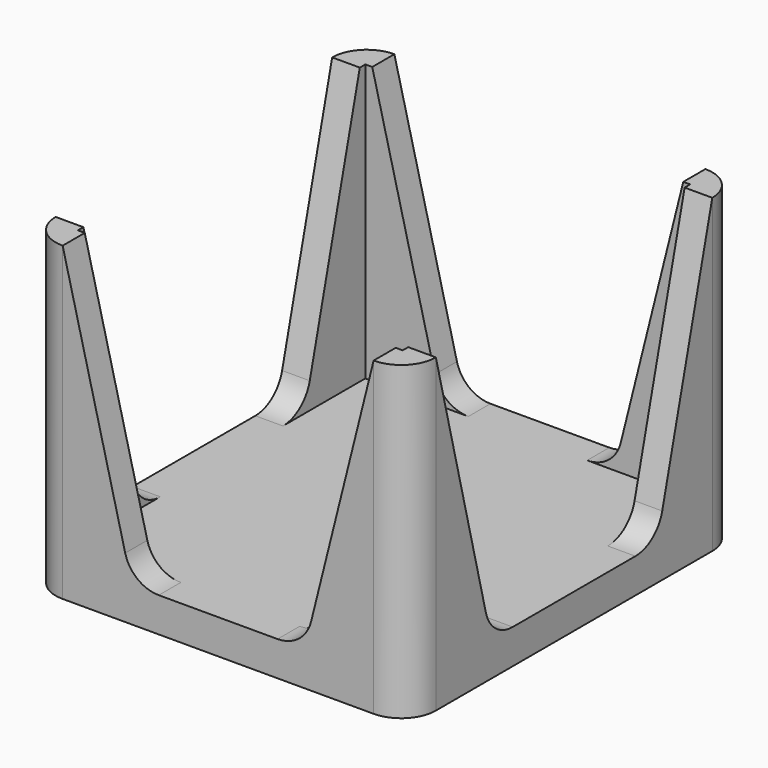
from build123d import *

# Parameters (mm, degrees)
F0_W         = 55
F0_H         = 60
F1_DEPTH     = 5
F3_DEPTH     = 40
F5_T4_DEPTH  = 211.7701999818
F5_T9_DEPTH  = 211.7701999818
F5_T14_DEPTH = 211.7701999818
F5_T19_DEPTH = 211.7701999818
F5_T24_DEPTH = 211.7701999818
F5_T29_DEPTH = 211.7701999818
F5_T34_DEPTH = 211.7701999818
F5_T39_DEPTH = 211.7701999818
F7_R         = 5
F8_R         = 5


# Not quite as in the source:
# - a fillet or chamfer that OpenCascade refuses, or shapes differently, is made with other operations: its cross-section is extruded or revolved along the edge and cut away or added
# - two fillets or chamfers of one size are made in one step
# - a feature of the source that left no trace in its solid (it failed there, or was rolled back) is left out


with BuildPart() as f1:
    # F0 (on Top) → F1 (new body)
    with BuildSketch(Plane.XY):
        Rectangle(F0_W, F0_H)
    extrude(amount=F1_DEPTH)

    # F2 (on face) → F3 (join)
    with BuildSketch(Plane.XY.offset(5)):
        Polygon((-23.5, 15), (-23.5, 26), (-12.5, 26), (-12.5, 30), (-27.5, 30), (-27.5, 15), align=None)
        Polygon((12.5, 30), (12.5, 26), (23.5, 26), (23.5, 15), (27.5, 15), (27.5, 30), align=None)
        Polygon((23.5, -26), (12.5, -26), (12.5, -30), (27.5, -30), (27.5, -15), (23.5, -15), align=None)
        Polygon((-23.5, -26), (-23.5, -15), (-27.5, -15), (-27.5, -30), (-12.5, -30), (-12.5, -26), align=None)
    extrude(amount=F3_DEPTH)

    # F5: chamfer of 10 x 40 on 8 edges, made by hand


with BuildPart() as f5_tool2:
    # F5_s3 → F5_t4 (new body)
    with BuildSketch(Plane.YZ.offset(-131.3850999909)):
        Polygon((15, 5), (25, 45), (15, 45), align=None)
    extrude(amount=F5_T4_DEPTH)

    split(bisect_by=Plane.XY.offset(5), keep=Keep.TOP)


with BuildPart() as f1_1:
    add(f1.part)

    # F5_t1: cut F5_tool2
    add(f5_tool2.part, mode=Mode.SUBTRACT)


with BuildPart() as f5_tool7:
    # F5_s8 → F5_t9 (new body)
    with BuildSketch(Plane.XZ.offset(-77.8850999909)):
        Polygon((22.5, 45), (12.5, 5), (12.5, 45), align=None)
    extrude(amount=F5_T9_DEPTH)

    split(bisect_by=Plane.XY.offset(5), keep=Keep.TOP)


with BuildPart() as f1_2:
    add(f1_1.part)

    # F5_t6: cut F5_tool7
    add(f5_tool7.part, mode=Mode.SUBTRACT)


with BuildPart() as f5_tool12:
    # F5_s13 → F5_t14 (new body)
    with BuildSketch(Plane.YZ.offset(-80.3850999909)):
        Polygon((15, 5), (25, 45), (15, 45), align=None)
    extrude(amount=F5_T14_DEPTH)

    split(bisect_by=Plane.XY.offset(5), keep=Keep.TOP)


with BuildPart() as f1_3:
    add(f1_2.part)

    # F5_t11: cut F5_tool12
    add(f5_tool12.part, mode=Mode.SUBTRACT)


with BuildPart() as f5_tool17:
    # F5_s18 → F5_t19 (new body)
    with BuildSketch(Plane.XZ.offset(-133.8850999909)):
        Polygon((12.5, 5), (22.5, 45), (12.5, 45), align=None)
    extrude(amount=F5_T19_DEPTH)

    split(bisect_by=Plane.XY.offset(5), keep=Keep.TOP)


with BuildPart() as f1_4:
    add(f1_3.part)

    # F5_t16: cut F5_tool17
    add(f5_tool17.part, mode=Mode.SUBTRACT)


with BuildPart() as f5_tool22:
    # F5_s23 → F5_t24 (new body)
    with BuildSketch(Plane.YZ.offset(131.3850999909)):
        Polygon((-25, 45), (-15, 5), (-15, 45), align=None)
    extrude(amount=-F5_T24_DEPTH)

    split(bisect_by=Plane.XY.offset(5), keep=Keep.TOP)


with BuildPart() as f1_5:
    add(f1_4.part)

    # F5_t21: cut F5_tool22
    add(f5_tool22.part, mode=Mode.SUBTRACT)


with BuildPart() as f5_tool27:
    # F5_s28 → F5_t29 (new body)
    with BuildSketch(Plane.XZ.offset(133.8850999909)):
        Polygon((-12.5, 5), (-22.5, 45), (-12.5, 45), align=None)
    extrude(amount=-F5_T29_DEPTH)

    split(bisect_by=Plane.XY.offset(5), keep=Keep.TOP)


with BuildPart() as f1_6:
    add(f1_5.part)

    # F5_t26: cut F5_tool27
    add(f5_tool27.part, mode=Mode.SUBTRACT)


with BuildPart() as f5_tool32:
    # F5_s33 → F5_t34 (new body)
    with BuildSketch(Plane.YZ.offset(80.3850999909)):
        Polygon((-15, 5), (-25, 45), (-15, 45), align=None)
    extrude(amount=-F5_T34_DEPTH)

    split(bisect_by=Plane.XY.offset(5), keep=Keep.TOP)


with BuildPart() as f1_7:
    add(f1_6.part)

    # F5_t31: cut F5_tool32
    add(f5_tool32.part, mode=Mode.SUBTRACT)


with BuildPart() as f5_tool37:
    # F5_s38 → F5_t39 (new body)
    with BuildSketch(Plane.XZ.offset(77.8850999909)):
        Polygon((-22.5, 45), (-12.5, 5), (-12.5, 45), align=None)
    extrude(amount=-F5_T39_DEPTH)

    split(bisect_by=Plane.XY.offset(5), keep=Keep.TOP)


with BuildPart() as f1_8:
    add(f1_7.part)

    # F5_t36: cut F5_tool37
    add(f5_tool37.part, mode=Mode.SUBTRACT)

    # F7
    f7_edges = [f1_8.edges().sort_by_distance(p)[0] for p in [
        (-27.5, -30, 22.5),
        (27.5, -30, 22.5),
        (27.5, 30, 22.5),
        (-27.5, 30, 22.5),
    ]]
    fillet(f7_edges, radius=F7_R)

    # F8
    f8_edges = [f1_8.edges().sort_by_distance(p)[0] for p in [
        (12.5, -28, 5),
        (12.5, 28, 5),
        (25.5, 15, 5),
        (-25.5, 15, 5),
        (-12.5, 28, 5),
        (-25.5, -15, 5),
        (-12.5, -28, 5),
        (25.5, -15, 5),
    ]]
    fillet(f8_edges, radius=F8_R)


solid = f1_8.part
